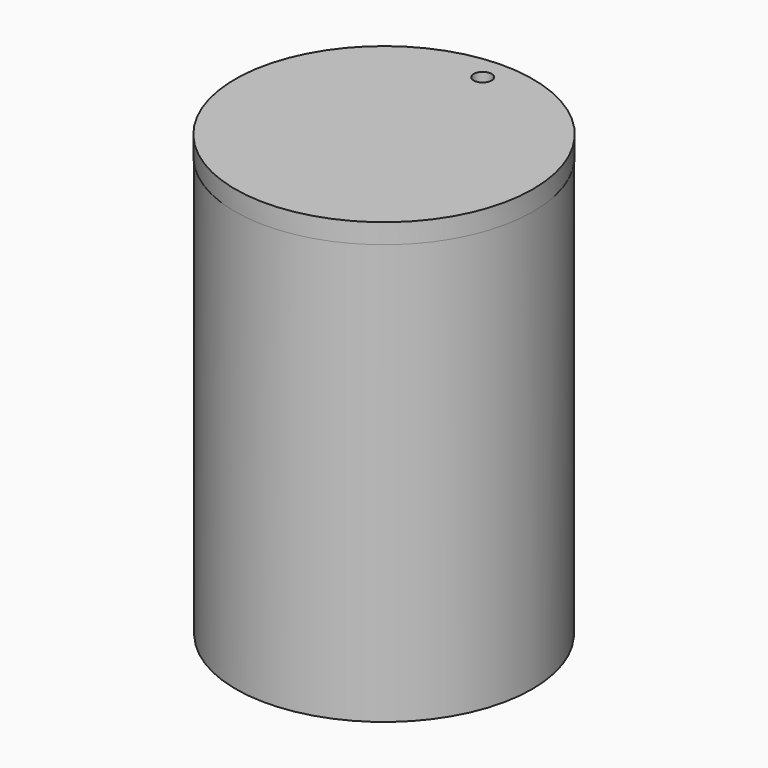
from build123d import *

# Parameters (mm, degrees)
F0_R           = 44.8176210425
F1_DEPTH       = 106.7643370479
F1_DEPTH_BACK  = 22.1521705389
F2_T           = -2.032
F3_R           = 3.7663248985
F4_DEPTH       = 59.9014814943
F5_START       = 91.4322212338
F2_FACE_R      = 42.7856210425
F5_DEPTH       = 13.5680139065
F6_T           = -1.524
F8_START       = 104.9826219678
F7_R           = 45.0292101327
F8_DEPTH       = 5.9961620718
F9_START       = 9.906
F5_FACE_R      = 42.7856210425
F9_DEPTH       = 15.494
F11_R          = 2.7160500701
F12_DEPTH      = 244.3860024214
F12_DEPTH_BACK = 45.8991546184


with BuildPart() as f1:
    # F0 (on Top) → F1 (new body, two sides)
    with BuildSketch(Plane.XY) as f1_sk:
        Circle(F0_R)
    extrude(amount=F1_DEPTH)
    extrude(f1_sk.sketch, amount=-F1_DEPTH_BACK)

    # F2
    f2_openings = [f1.faces().sort_by_distance(p)[0] for p in [
        (0, 0, 106.764337),
    ]]
    offset(amount=F2_T, openings=f2_openings)

    # F3 (on Front) → F4 (cut)
    with BuildSketch(Plane.XZ):
        with Locations((0, 89.9693667889)):
            Circle(F3_R)
    extrude(amount=-F4_DEPTH, mode=Mode.SUBTRACT)


with BuildPart() as f5:
    # F2_face (on face) → F5 (new body)
    with BuildSketch(Plane.XY.offset(-20.1201705389).offset(F5_START)):
        Circle(F2_FACE_R)
    extrude(amount=F5_DEPTH)

    # F6
    f6_openings = [f5.faces().sort_by_distance(p)[0] for p in [
        (0, 0, 71.312051),
    ]]
    offset(amount=F6_T, openings=f6_openings)


with BuildPart() as f8:
    # F7 (on Top) → F8 (new body)
    with BuildSketch(Plane.XY.offset(F8_START)):
        Circle(F7_R)
    extrude(amount=F8_DEPTH)

    # F5_face (on face) → F9 (join)
    with BuildSketch(Plane.XY.offset(84.8800646014).offset(F9_START)):
        Circle(F5_FACE_R)
    extrude(amount=F9_DEPTH)

    # F11 (on Top) → F12 (cut, two sides)
    with BuildSketch(Plane.XY) as f12_sk:
        with Locations((0, 37.2846573591)):
            Circle(F11_R)
    extrude(amount=F12_DEPTH, mode=Mode.SUBTRACT)
    extrude(f12_sk.sketch, amount=-F12_DEPTH_BACK, mode=Mode.SUBTRACT)


solid = Compound([f1.part, f8.part])
